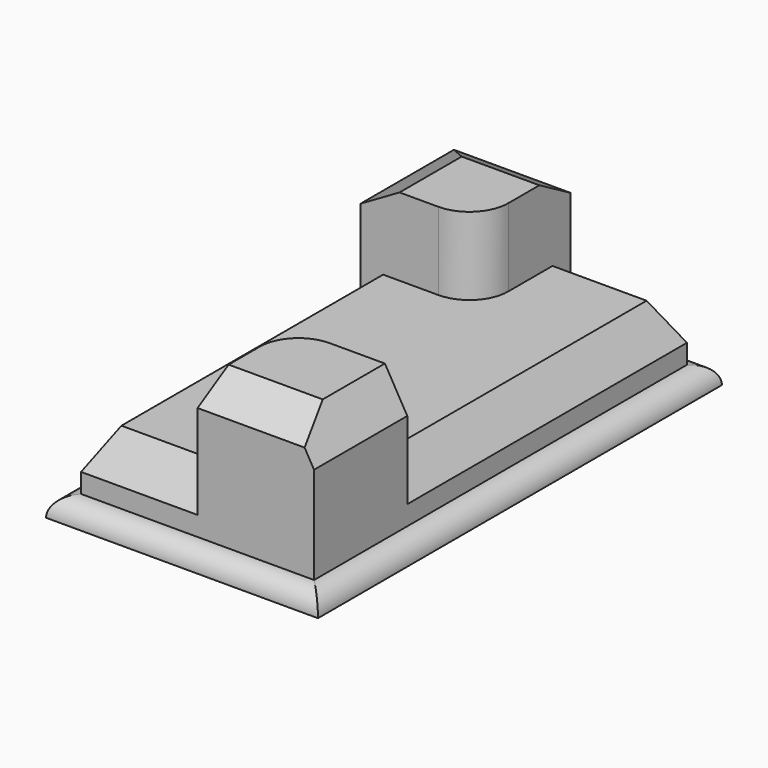
from build123d import *

# Parameters (mm, degrees)
F0_W        = 88.9
F0_H        = 165.1
F1_DEPTH    = 6.35
F2_DEPTH    = 25.4
F3_DEPTH    = 50.8
F4_R        = 6.34999
F5_C1_SIZE2 = 12.7
F5_C1_SIZE  = 7.3323484187
F5_C2_SIZE2 = 7.3323484187
F5_C2_SIZE  = 12.7
F5_C3_SIZE2 = 7.3323484187
F5_C3_SIZE  = 12.7
F5_C4_SIZE2 = 7.3323484187
F5_C4_SIZE  = 12.7
F5_C5_SIZE2 = 7.3323484187
F5_C5_SIZE  = 12.7
F5_C6_SIZE2 = 7.3323484187
F5_C6_SIZE  = 12.7
F5_C7_SIZE2 = 12.7
F5_C7_SIZE  = 7.3323484187
F6_SIZE2    = 7.3323484187
F6_SIZE     = 12.7


# Not quite as in the source:
# - a fillet or chamfer is up to 0.001 mm smaller than in the source, because OpenCascade refuses the exact size


with BuildPart() as f1:
    # F0 (on Top) → F1 (new body)
    with BuildSketch(Plane.XY):
        Rectangle(F0_W, F0_H)
        Polygon((-38.1, 38.1), (-38.1, 76.2), (0, 76.2), (38.1, 76.2), (38.1, -38.1), (38.1, -76.2), (0, -76.2), (-38.1, -76.2), align=None, mode=Mode.SUBTRACT)
    extrude(amount=F1_DEPTH)

    # F0 (on Top) → F2 (join)
    with BuildSketch(Plane.XY):
        with BuildLine():
            Line((38.1, 76.2), (0, 76.2))
            Line((0, 76.2), (0, 50.8))
            ThreePointArc((0, 50.8), (-3.7197438789, 41.8197438789), (-12.7, 38.1))
            Line((-12.7, 38.1), (-38.1, 38.1))
            Line((-38.1, 38.1), (-38.1, -76.2))
            Line((-38.1, -76.2), (0, -76.2))
            Line((0, -76.2), (0, -50.8))
            ThreePointArc((0, -50.8), (3.7197438789, -41.8197438789), (12.7, -38.1))
            Line((12.7, -38.1), (38.1, -38.1))
            Line((38.1, -38.1), (38.1, 76.2))
        make_face()
    extrude(amount=F2_DEPTH)

    # F0 (on Top) → F3 (join)
    with BuildSketch(Plane.XY):
        with BuildLine():
            Line((38.1, -76.2), (38.1, -38.1))
            Line((38.1, -38.1), (12.7, -38.1))
            ThreePointArc((12.7, -38.1), (3.7197438789, -41.8197438789), (0, -50.8))
            Line((0, -50.8), (0, -76.2))
            Line((0, -76.2), (38.1, -76.2))
        make_face()
        with BuildLine():
            Line((0, 76.2), (-38.1, 76.2))
            Line((-38.1, 76.2), (-38.1, 38.1))
            Line((-38.1, 38.1), (-12.7, 38.1))
            ThreePointArc((-12.7, 38.1), (-3.7197438789, 41.8197438789), (0, 50.8))
            Line((0, 50.8), (0, 76.2))
        make_face()
    extrude(amount=F3_DEPTH)

    # F4 (radius 6.35 in the source; OpenCascade refuses exactly that, so slightly less here)
    f4_edges = [f1.edges().sort_by_distance(p)[0] for p in [
        (0, -82.55, 6.35),
        (44.45, 0, 6.35),
        (0, 82.55, 6.35),
        (-44.45, 0, 6.35),
    ]]
    fillet(f4_edges, radius=F4_R)

    # F5: chamfer of 12.7 x 7.3323484187 on 7 edges, made by hand

    # F5_c1
    f5_c1_edges = [f1.edges().sort_by_distance(p)[0] for p in [
        (-38.1, 57.15, 50.8),
    ]]
    f5_c1_side = f1.faces().sort_by_distance((-38.1, 57.15, 50.6533530316))[0]
    chamfer(f5_c1_edges, length=F5_C1_SIZE, length2=F5_C1_SIZE2, reference=f5_c1_side)

    # F5_c2
    f5_c2_edges = [f1.edges().sort_by_distance(p)[0] for p in [
        (-38.1, -19.05, 25.4),
    ]]
    f5_c2_side = f1.faces().sort_by_distance((-38.1, -19.05, 25.2533530316))[0]
    chamfer(f5_c2_edges, length=F5_C2_SIZE, length2=F5_C2_SIZE2, reference=f5_c2_side)

    # F5_c3
    f5_c3_edges = [f1.edges().sort_by_distance(p)[0] for p in [
        (19.05, 76.2, 25.4),
    ]]
    f5_c3_side = f1.faces().sort_by_distance((19.05, 76.2, 25.2533530316))[0]
    chamfer(f5_c3_edges, length=F5_C3_SIZE, length2=F5_C3_SIZE2, reference=f5_c3_side)

    # F5_c4
    f5_c4_edges = [f1.edges().sort_by_distance(p)[0] for p in [
        (38.1, -57.15, 50.8),
    ]]
    f5_c4_side = f1.faces().sort_by_distance((38.1, -57.15, 50.6533530316))[0]
    chamfer(f5_c4_edges, length=F5_C4_SIZE, length2=F5_C4_SIZE2, reference=f5_c4_side)

    # F5_c5
    f5_c5_edges = [f1.edges().sort_by_distance(p)[0] for p in [
        (38.1, 15.3838257906, 25.4),
    ]]
    f5_c5_side = f1.faces().sort_by_distance((38.1, 15.3838257906, 25.2533530316))[0]
    chamfer(f5_c5_edges, length=F5_C5_SIZE, length2=F5_C5_SIZE2, reference=f5_c5_side)

    # F5_c6
    f5_c6_edges = [f1.edges().sort_by_distance(p)[0] for p in [
        (-15.3838257906, -76.2, 25.4),
    ]]
    f5_c6_side = f1.faces().sort_by_distance((-15.3838257906, -76.2, 25.2533530316))[0]
    chamfer(f5_c6_edges, length=F5_C6_SIZE, length2=F5_C6_SIZE2, reference=f5_c6_side)

    # F5_c7
    f5_c7_edges = [f1.edges().sort_by_distance(p)[0] for p in [
        (15.3838257906, -76.2, 50.8),
    ]]
    f5_c7_side = f1.faces().sort_by_distance((15.3838257906, -76.2, 50.6533530316))[0]
    chamfer(f5_c7_edges, length=F5_C7_SIZE, length2=F5_C7_SIZE2, reference=f5_c7_side)

    # F6
    f6_edges = [f1.edges().sort_by_distance(p)[0] for p in [
        (-12.7, 76.2, 50.8),
    ]]
    f6_side = f1.faces().sort_by_distance((-13.065864, 57.751409, 50.8))[0]
    chamfer(f6_edges, length=F6_SIZE, length2=F6_SIZE2, reference=f6_side)


solid = f1.part
